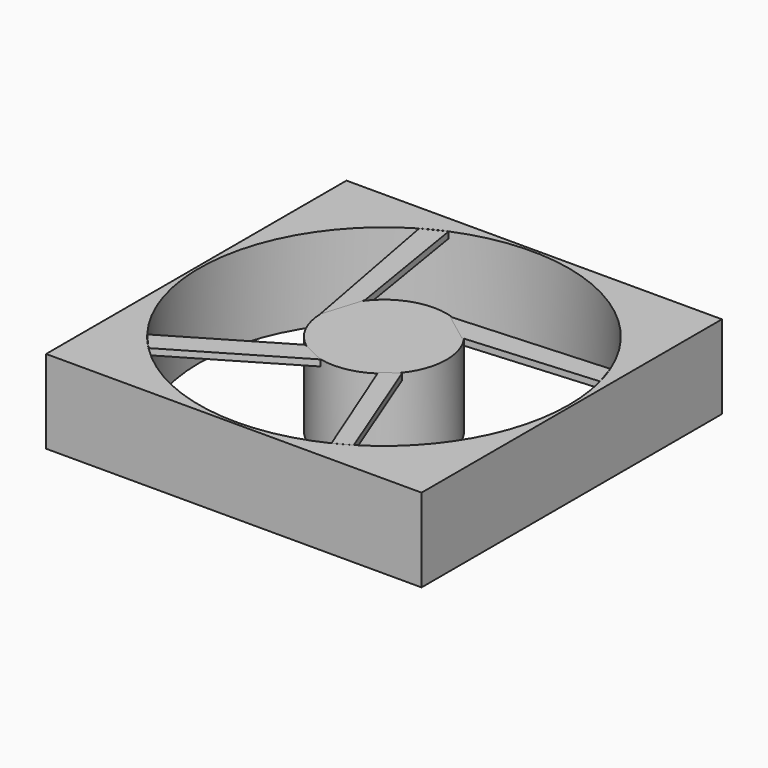
from build123d import *

# Parameters (mm, degrees)
F0_W     = 9
F0_H     = 9
F1_DEPTH = 2
F2_R     = 4.43316962
F2_R_2   = 1.5
F3_DEPTH = 3
F5_DEPTH = 0.15
F6_DEPTH = 0.15


# Not quite as in the source:
# - a feature of the source that left no trace in its solid (it failed there, or was rolled back) is left out
# - the program builds the solid bodies; features that only make, move or delete a surface that nothing else refers to are left out


with BuildPart() as f1:
    # F0 (on Top) → F1 (new body)
    with BuildSketch(Plane.XY):
        with Locations((-4.5, 4.5)):
            Rectangle(F0_W, F0_H)
    extrude(amount=F1_DEPTH)

    # F2 (on face) → F3 (cut)
    with BuildSketch(Plane.XY.offset(2)):
        with Locations((-4.5, 4.5)):
            Circle(F2_R)
        with Locations((-4.5, 4.5)):
            Circle(F2_R_2, mode=Mode.SUBTRACT)
    extrude(amount=-F3_DEPTH, mode=Mode.SUBTRACT)

    # F4 (on face) → F5 (cut)
    with BuildSketch(Plane.XY.offset(2)):
        Polygon((-6.7244199271, 8.3347032307), (-6.0038217343, 4.4680763967), (-5.7035977952, 5.4315547459), (-6.2189687337, 8.5863356901), align=None)
        Polygon((-0.3756961864, 6.1257647226), (-4.0373285301, 5.9030898847), (-3.3286872786, 5.3683454171), (-0.2075215072, 5.6079807167), align=None)
        Polygon((-4.849715769, 3.0361308041), (-5.4445206188, 3.3202320337), (-8.017316279, 1.8015784108), (-7.6516059208, 1.3822487271), align=None)
        Polygon((-3.3131770324, 3.5631777719), (-3.6769588478, 3.2967031002), (-2.5675997073, 0.510160155), (-2.1946810339, 0.7133791655), align=None)
    extrude(amount=-F5_DEPTH, mode=Mode.SUBTRACT)


with BuildPart() as f6:
    # F4 (on face) → F6 (new body)
    with BuildSketch(Plane.XY.offset(2)):
        Polygon((-6.7244199271, 8.3347032307), (-6.0038217343, 4.4680763967), (-5.7035977952, 5.4315547459), (-6.2189687337, 8.5863356901), align=None)
    extrude(amount=-F6_DEPTH)


with BuildPart() as f6b:
    # F4 (on face) → F6, piece 2 (new body)
    with BuildSketch(Plane.XY.offset(2)):
        Polygon((-0.3756961864, 6.1257647226), (-4.0373285301, 5.9030898847), (-3.3286872786, 5.3683454171), (-0.2075215072, 5.6079807167), align=None)
    extrude(amount=-F6_DEPTH)


with BuildPart() as f6c:
    # F4 (on face) → F6, piece 3 (new body)
    with BuildSketch(Plane.XY.offset(2)):
        Polygon((-4.849715769, 3.0361308041), (-5.4445206188, 3.3202320337), (-8.017316279, 1.8015784108), (-7.6516059208, 1.3822487271), align=None)
    extrude(amount=-F6_DEPTH)


with BuildPart() as f6d:
    # F4 (on face) → F6, piece 4 (new body)
    with BuildSketch(Plane.XY.offset(2)):
        Polygon((-3.3131770324, 3.5631777719), (-3.6769588478, 3.2967031002), (-2.5675997073, 0.510160155), (-2.1946810339, 0.7133791655), align=None)
    extrude(amount=-F6_DEPTH)


solid = Compound([f1.part, f6.part, f6b.part, f6c.part, f6d.part])
